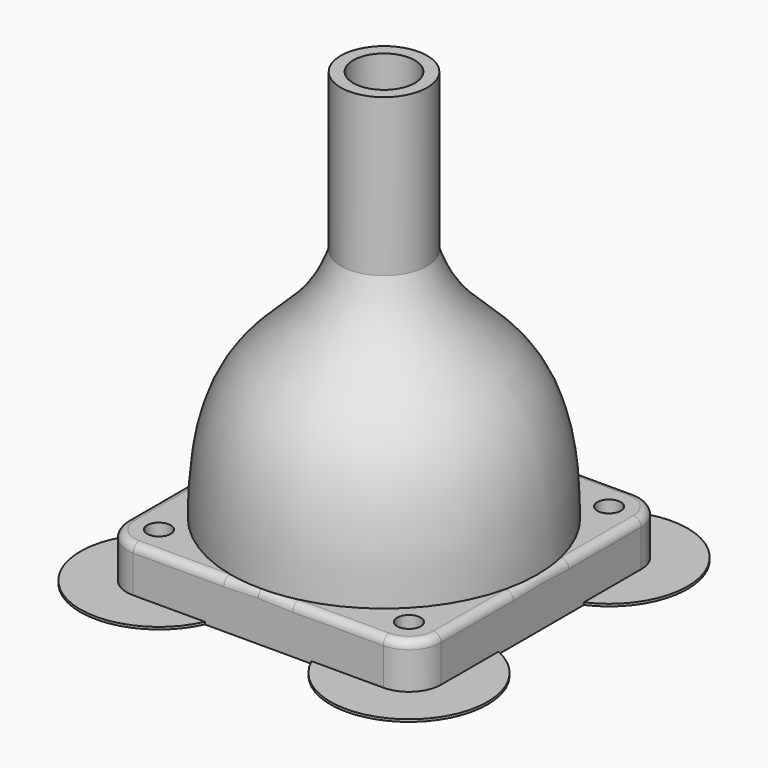
from build123d import *

# Parameters (mm, degrees)
F0_R     = 1.5
F0_R_2   = 18
F1_DEPTH = 6
F0_R_3   = 12
F5_REACH = 65.9117488974
F6_R     = 1
F8_DEPTH = 0.3


# Not quite as in the source:
# - ends of sketch curves that miss each other by under 0.0002 mm in the source are joined
# - the dataset's text gives a spline's control points without its knots; the knots are read off the source's solid


with BuildPart() as f1:
    # F0 (on Top) → F1 (new body)
    with BuildSketch(Plane.XY):
        with BuildLine():
            Line((15.9099025767, 20), (-15.9099025767, 20))
            ThreePointArc((-15.9099025767, 20), (-18.8020382004, 18.8020382004), (-20, 15.9099025767))
            Line((-20, 15.9099025767), (-20, -15.9099025767))
            ThreePointArc((-20, -15.9099025767), (-18.8020382004, -18.8020382004), (-15.9099025767, -20))
            Line((-15.9099025767, -20), (15.9099025767, -20))
            ThreePointArc((15.9099025767, -20), (18.8020382004, -18.8020382004), (20, -15.9099025767))
            Line((20, -15.9099025767), (20, 15.9099025767))
            ThreePointArc((20, 15.9099025767), (18.8020382004, 18.8020382004), (15.9099025767, 20))
        make_face()
        with Locations((-15.9099025767, -15.9099025767)):
            Circle(F0_R, mode=Mode.SUBTRACT)
        with Locations((15.9099025767, -15.9099025767)):
            Circle(F0_R, mode=Mode.SUBTRACT)
        with Locations((-15.9099025767, 15.9099025767)):
            Circle(F0_R, mode=Mode.SUBTRACT)
        Circle(F0_R_2, mode=Mode.SUBTRACT)
        with Locations((15.9099025767, 15.9099025767)):
            Circle(F0_R, mode=Mode.SUBTRACT)
    extrude(amount=F1_DEPTH)

    # F2 (on Right) → F3 (revolve)
    with BuildSketch(Plane.YZ):
        with BuildLine():
            Line((-19.5, 6), (-18, 6))
            add(Edge.make_bspline(
                [(-18, 6), (-18.0000000001, 27.6965421784), (-8.279467036, 22.2953179595), (-3.9214516831, 36)],
                knots=[0, 0, 0, 0, 36.6527581606, 36.6527581606, 36.6527581606, 36.6527581606], degree=3))
            Line((-3.9214516831, 36), (-3.9214516831, 56))
            Line((-3.9214516831, 56), (-5.5, 56))
            Line((-5.5, 56), (-5.5, 36))
            add(Edge.make_bspline(
                [(-19.5, 6), (-19.5, 9.3312793591), (-19.1645857225, 13.4358860925), (-18.164345948, 17.6087871702), (-17.1644902836, 20.1948148106), (-15.9543392588, 22.3267545538), (-14.5971497125, 24.0868775249), (-13.1708159242, 25.5729079811), (-11.7428886797, 26.9014988935), (-10.3589447723, 28.1943988027), (-9.0438163865, 29.5716652795), (-7.8069298643, 31.1579880004), (-6.6551252979, 33.0905671825), (-5.9096418293, 34.8169074272), (-5.5436229413, 35.8710078247), (-5.5, 36)],
                knots=[0, 0, 0, 0, 0.125, 0.1875, 0.25, 0.3125, 0.375, 0.4375, 0.5, 0.5625, 0.625, 0.6875, 0.75, 0.8125, 0.8210592996, 0.8210592996, 0.8210592996, 0.8210592996], degree=3))
        make_face()
    revolve(axis=Axis((0, 0, 13.5), (0, 0, -1)))



with BuildPart() as f1b:
    # F0 (on Top) → F1, piece 2 (new body)
    with BuildSketch(Plane.XY):
        Circle(F0_R_3)
    extrude(amount=F1_DEPTH)

    # F2 (on Right) → F3, piece 2 (revolve)
    with BuildSketch(Plane.YZ):
        with BuildLine():
            add(Edge.make_bspline(
                [(-12, 6), (-12, 12.1178685978), (0, 12.1178685978), (0, 21)],
                knots=[0, 0, 0, 0, 19.2093727123, 19.2093727123, 19.2093727123, 19.2093727123], degree=3))
            Line((-12, 6), (0, 6))
            Line((0, 6), (0, 21))
        make_face()
    revolve(axis=Axis((0, 0, 13.5), (0, 0, -1)))


with BuildPart() as f1_1:
    add(f1.part)

    add(f1b.part)  # F5 merges F1b
    f5_end = f1_1.faces().sort_by_distance((0, 12.5949815989, 23.9969475517))[0]
    # F4 (on Top) → F5 (join, up to a face of the model that its end follows)
    with BuildSketch(Plane.XY):
        with BuildLine():
            Line((-0.375, -8.7419605925), (-0.375, -17.9960933261))
            ThreePointArc((-0.375, -17.9960933261), (0, -18), (0.375, -17.9960933261))
            Line((0.375, -17.9960933261), (0.375, -8.7419605925))
            ThreePointArc((0.375, -8.7419605925), (0, -8.75), (-0.375, -8.7419605925))
        make_face()
        with BuildLine():
            Line((7.7582599519, 4.0462207698), (15.7725739892, 8.6732871366))
            ThreePointArc((15.7725739892, 8.6732871366), (15.5884572681, 9), (15.3975739892, 9.3228061894))
            Line((15.3975739892, 9.3228061894), (7.3832599519, 4.6957398226))
            ThreePointArc((7.3832599519, 4.6957398226), (7.5777222831, 4.375), (7.7582599519, 4.0462207698))
        make_face()
        with BuildLine():
            Line((-7.3832599519, 4.6957398226), (-15.3975739892, 9.3228061894))
            ThreePointArc((-15.3975739892, 9.3228061894), (-15.5884572681, 9), (-15.7725739892, 8.6732871366))
            Line((-15.7725739892, 8.6732871366), (-7.7582599519, 4.0462207698))
            ThreePointArc((-7.7582599519, 4.0462207698), (-7.5777222831, 4.375), (-7.3832599519, 4.6957398226))
        make_face()
    f5_long = extrude(amount=F5_REACH, mode=Mode.PRIVATE)
    add(split(f5_long, bisect_by=f5_end, keep=Keep.TOP, mode=Mode.PRIVATE))

    # F6
    f6_edges = [f1_1.edges().sort_by_distance(p)[0] for p in [
        (-20, 0, 6),
        (18.802038, 18.802038, 6),
        (18.802038, -18.802038, 6),
        (-18.802038, 18.802038, 6),
        (-18.802038, -18.802038, 6),
    ]]
    fillet(f6_edges, radius=F6_R)

    # F7 (on face) → F8 (join)
    with BuildSketch(Plane(origin=(0, 0, 0), x_dir=(1, 0, 0), z_dir=(0, 0, -1))):
        with BuildLine():
            ThreePointArc((6.7846024135, -20), (22.9809703886, -22.9809703886), (20, -6.7846024135))
            Line((20, -6.7846024135), (20, -15.9099025767))
            ThreePointArc((20, -15.9099025767), (18.8020382004, -18.8020382004), (15.9099025767, -20))
            Line((15.9099025767, -20), (6.7846024135, -20))
        make_face()
        with BuildLine():
            Line((-20, -15.9099025767), (-20, -6.7846024135))
            ThreePointArc((-20, -6.7846024135), (-22.9809703886, -22.9809703886), (-6.7846024135, -20))
            Line((-6.7846024135, -20), (-15.9099025767, -20))
            ThreePointArc((-15.9099025767, -20), (-18.8020382004, -18.8020382004), (-20, -15.9099025767))
        make_face()
        with BuildLine():
            Line((-15.9099025767, 20), (-6.7846024135, 20))
            ThreePointArc((-6.7846024135, 20), (-22.9809703886, 22.9809703886), (-20, 6.7846024135))
            Line((-20, 6.7846024135), (-20, 15.9099025767))
            ThreePointArc((-20, 15.9099025767), (-18.8020382004, 18.8020382004), (-15.9099025767, 20))
        make_face()
        with BuildLine():
            ThreePointArc((20, 6.7846024135), (22.9809703886, 22.9809703886), (6.7846024135, 20))
            Line((6.7846024135, 20), (15.9099025767, 20))
            ThreePointArc((15.9099025767, 20), (18.8020382004, 18.8020382004), (20, 15.9099025767))
            Line((20, 15.9099025767), (20, 6.7846024135))
        make_face()
    extrude(amount=-F8_DEPTH)


solid = f1_1.part
